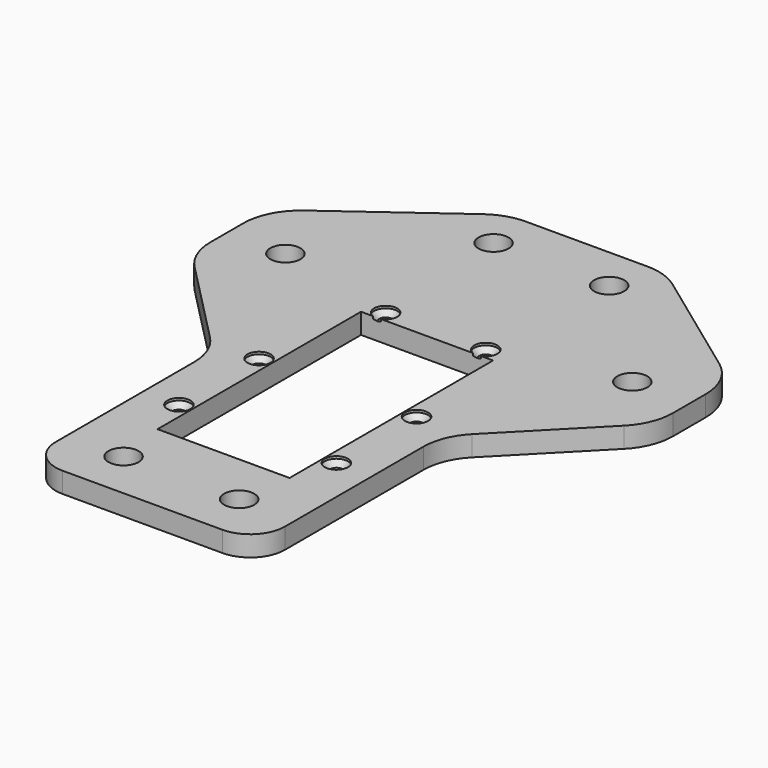
from build123d import *

# Parameters (mm, degrees)
F0_R         = 3.302
F0_R_2       = 1.397
F1_DEPTH     = 4.4958
F3_R         = 2.54
F4_DEPTH     = 0.381
F5_S5_R      = 2.54
F5_T6_DEPTH  = 5
F5_S11_R     = 2.54
F5_T12_DEPTH = 5
F5_S17_R     = 2.54
F5_T18_DEPTH = 5
F5_S23_R     = 2.54
F5_T24_DEPTH = 5
F5_S29_R     = 2.54
F5_T30_DEPTH = 5
F5_S35_R     = 2.54
F5_T36_DEPTH = 5


# Not quite as in the source:
# - a fillet or chamfer that OpenCascade refuses, or shapes differently, is made with other operations: its cross-section is extruded or revolved along the edge and cut away or added


with BuildPart() as f1:
    # F0 (on Top) → F1 (new body)
    with BuildSketch(Plane.XY):
        with BuildLine():
            Line((0, 71.7569190334), (-13.3202167361, 71.7569190334))
            ThreePointArc((-13.3202167361, 71.7569190334), (-17.2583195593, 71.1309136563), (-20.8081903285, 69.3146113411))
            Line((-20.8081903285, 69.3146113411), (-45.5879735924, 51.2257120897))
            ThreePointArc((-45.5879735924, 51.2257120897), (-49.4222626852, 46.7209640446), (-50.8, 40.968019782))
            Line((-50.8, 40.968019782), (-50.8, 31.9697443563))
            ThreePointArc((-50.8, 31.9697443563), (-49.8574337411, 27.1684162251), (-47.1696453822, 23.0797762663))
            Line((-47.1696453822, 23.0797762663), (-28.8017546178, 4.3406476252))
            ThreePointArc((-28.8017546178, 4.3406476252), (-26.1139662589, 0.2520076664), (-25.1714, -4.5493204647))
            Line((-25.1714, -4.5493204647), (-25.1714, -42.5430809666))
            ThreePointArc((-25.1714, -42.5430809666), (-22.9395536726, -47.9312346392), (-17.5514, -50.1630809666))
            Line((-17.5514, -50.1630809666), (0, -50.1630809666))
            Line((0, -50.1630809666), (0, -27.9380809666))
            Line((0, -27.9380809666), (-14.5034, -27.9380809666))
            Line((-14.5034, -27.9380809666), (-14.5034, 27.9419190334))
            Line((-14.5034, 27.9419190334), (0, 27.9419190334))
            Line((0, 27.9419190334), (0, 71.7569190334))
        make_face()
        with Locations((-12.7, -39.5204809666)):
            Circle(F0_R, mode=Mode.SUBTRACT)
        with Locations((-17.2974, -18.5654809666)):
            Circle(F0_R_2, mode=Mode.SUBTRACT)
        with Locations((-17.2974, 3.4309190334)):
            Circle(F0_R_2, mode=Mode.SUBTRACT)
        with Locations((-38.1, 36.6795190334)):
            Circle(F0_R, mode=Mode.SUBTRACT)
        with Locations((-10.9982, 30.3231690334)):
            Circle(F0_R_2, mode=Mode.SUBTRACT)
        with Locations((-12.7, 62.0795190334)):
            Circle(F0_R, mode=Mode.SUBTRACT)
    extrude(amount=F1_DEPTH)

    # F2: F1 across face


with BuildPart() as f1_1:
    add(f1.part)
    add(f1.part.mirror(Plane(origin=(0, 49.8494190334, 2.2479), x_dir=(0, 1, 0), z_dir=(1, 0, 0))))

    # F3 (on face) → F4 (cut)
    with BuildSketch(Plane.XY.offset(4.4958)):
        with Locations((-10.9982, 30.3231690334)):
            Circle(F3_R)
        with Locations((-17.2974, 3.4309190334)):
            Circle(F3_R)
        with Locations((-17.2974, -18.5654809666)):
            Circle(F3_R)
        with Locations((10.9982, 30.3231690334)):
            Circle(F3_R)
        with Locations((17.2974, 3.4309190334)):
            Circle(F3_R)
        with Locations((17.2974, -18.5654809666)):
            Circle(F3_R)
    extrude(amount=-F4_DEPTH, mode=Mode.SUBTRACT)

    # F5: chamfer of 1.27 on 6 edges, made by hand


with BuildPart() as f5_tool2:
    # F5_s3 → F5_t4 (revolve)
    with BuildSketch(Plane.XZ.offset(-30.3231690334)):
        Polygon((-8.3312, 4.1148), (-9.6012, 2.8448), (-9.6012, 4.1148), align=None)
    revolve(axis=Axis((-10.9982, 30.3231690334, 4.1148), (0, 0, -1)))

    # F5_s5 → F5_t6 (intersect, symmetric)
    with BuildSketch(Plane.XY.offset(3.5)):
        with Locations((-10.9982, 30.3231690334)):
            Circle(F5_S5_R)
    extrude(amount=F5_T6_DEPTH, both=True, mode=Mode.INTERSECT)


with BuildPart() as f1_2:
    add(f1_1.part)

    # F5_t1: cut F5_tool2
    add(f5_tool2.part, mode=Mode.SUBTRACT)


with BuildPart() as f5_tool8:
    # F5_s9 → F5_t10 (revolve)
    with BuildSketch(Plane.XZ.offset(-30.3231690334)):
        Polygon((8.3312, 4.1148), (9.6012, 2.8448), (9.6012, 4.1148), align=None)
    revolve(axis=Axis((10.9982, 30.3231690334, 4.1148), (0, 0, -1)))

    # F5_s11 → F5_t12 (intersect, symmetric)
    with BuildSketch(Plane.XY.offset(3.5)):
        with Locations((10.9982, 30.3231690334)):
            Circle(F5_S11_R)
    extrude(amount=F5_T12_DEPTH, both=True, mode=Mode.INTERSECT)


with BuildPart() as f1_3:
    add(f1_2.part)

    # F5_t7: cut F5_tool8
    add(f5_tool8.part, mode=Mode.SUBTRACT)


with BuildPart() as f5_tool14:
    # F5_s15 → F5_t16 (revolve)
    with BuildSketch(Plane.XZ.offset(-3.4309190334)):
        Polygon((-14.6304, 4.1148), (-15.9004, 2.8448), (-15.9004, 4.1148), align=None)
    revolve(axis=Axis((-17.2974, 3.4309190334, 4.1148), (0, 0, -1)))

    # F5_s17 → F5_t18 (intersect, symmetric)
    with BuildSketch(Plane.XY.offset(3.5)):
        with Locations((-17.2974, 3.4309190334)):
            Circle(F5_S17_R)
    extrude(amount=F5_T18_DEPTH, both=True, mode=Mode.INTERSECT)


with BuildPart() as f1_4:
    add(f1_3.part)

    # F5_t13: cut F5_tool14
    add(f5_tool14.part, mode=Mode.SUBTRACT)


with BuildPart() as f5_tool20:
    # F5_s21 → F5_t22 (revolve)
    with BuildSketch(Plane.XZ.offset(-3.4309190334)):
        Polygon((14.6304, 4.1148), (15.9004, 2.8448), (15.9004, 4.1148), align=None)
    revolve(axis=Axis((17.2974, 3.4309190334, 4.1148), (0, 0, -1)))

    # F5_s23 → F5_t24 (intersect, symmetric)
    with BuildSketch(Plane.XY.offset(3.5)):
        with Locations((17.2974, 3.4309190334)):
            Circle(F5_S23_R)
    extrude(amount=F5_T24_DEPTH, both=True, mode=Mode.INTERSECT)


with BuildPart() as f1_5:
    add(f1_4.part)

    # F5_t19: cut F5_tool20
    add(f5_tool20.part, mode=Mode.SUBTRACT)


with BuildPart() as f5_tool26:
    # F5_s27 → F5_t28 (revolve)
    with BuildSketch(Plane.XZ.offset(18.5654809666)):
        Polygon((-14.6304, 4.1148), (-15.9004, 2.8448), (-15.9004, 4.1148), align=None)
    revolve(axis=Axis((-17.2974, -18.5654809666, 4.1148), (0, 0, -1)))

    # F5_s29 → F5_t30 (intersect, symmetric)
    with BuildSketch(Plane.XY.offset(3.5)):
        with Locations((-17.2974, -18.5654809666)):
            Circle(F5_S29_R)
    extrude(amount=F5_T30_DEPTH, both=True, mode=Mode.INTERSECT)


with BuildPart() as f1_6:
    add(f1_5.part)

    # F5_t25: cut F5_tool26
    add(f5_tool26.part, mode=Mode.SUBTRACT)


with BuildPart() as f5_tool32:
    # F5_s33 → F5_t34 (revolve)
    with BuildSketch(Plane.XZ.offset(18.5654809666)):
        Polygon((14.6304, 4.1148), (15.9004, 2.8448), (15.9004, 4.1148), align=None)
    revolve(axis=Axis((17.2974, -18.5654809666, 4.1148), (0, 0, -1)))

    # F5_s35 → F5_t36 (intersect, symmetric)
    with BuildSketch(Plane.XY.offset(3.5)):
        with Locations((17.2974, -18.5654809666)):
            Circle(F5_S35_R)
    extrude(amount=F5_T36_DEPTH, both=True, mode=Mode.INTERSECT)


with BuildPart() as f1_7:
    add(f1_6.part)

    # F5_t31: cut F5_tool32
    add(f5_tool32.part, mode=Mode.SUBTRACT)


solid = f1_7.part
